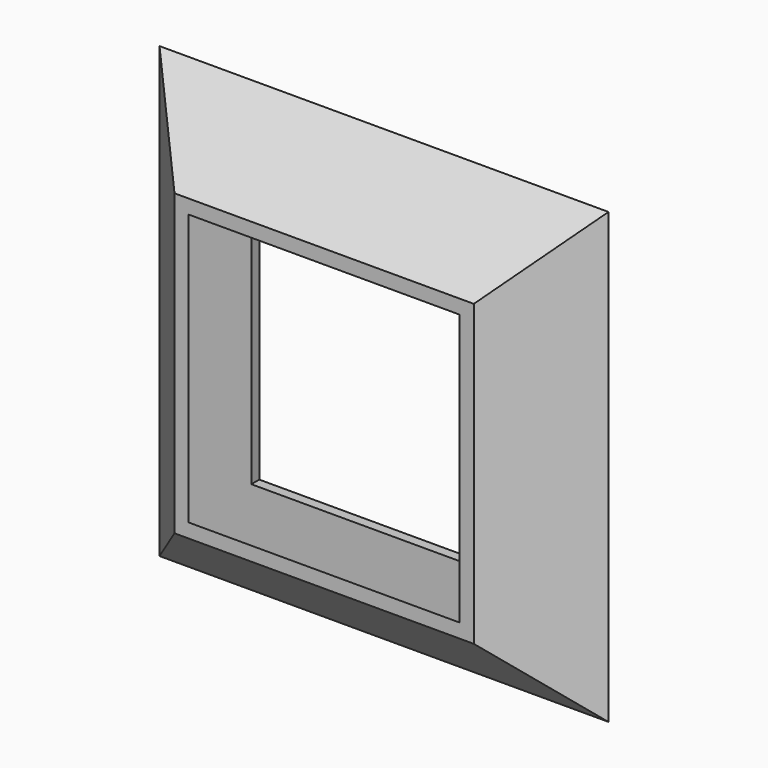
from build123d import *

# Parameters (mm, degrees)
F0_W        = 127
F0_H        = 127
F1_DEPTH    = 19.05
F2_T1_DEPTH = 257.6414957887
F2_T3_DEPTH = 257.6414957887
F3_T        = -2.54
F4_W        = 63.5
F4_H        = 63.5
F5_DEPTH    = 25.4


# Not quite as in the source:
# - a fillet or chamfer that OpenCascade refuses, or shapes differently, is made with other operations: its cross-section is extruded or revolved along the edge and cut away or added


with BuildPart() as f1:
    # F0 (on Front) → F1 (new body)
    with BuildSketch(Plane.XZ):
        with Locations((-51.5997745097, 45.6864875067)):
            Rectangle(F0_W, F0_H)
    extrude(amount=F1_DEPTH)

    # F2: chamfer of 25.4 on 4 edges, made by hand

    # F2_s2 → F2_t1 (cut)
    with BuildSketch(Plane.XY.offset(-83.1342603876)):
        Polygon((11.9002254903, 6.35), (-13.4997745097, -19.05), (11.9002254903, -19.05), align=None)
        Polygon((-115.0997745097, 6.35), (-89.6997745097, -19.05), (-115.0997745097, -19.05), align=None)
    extrude(amount=F2_T1_DEPTH, mode=Mode.SUBTRACT)

    # F2_s4 → F2_t3 (cut)
    with BuildSketch(Plane.YZ.offset(-180.420522404)):
        Polygon((6.35, 109.1864875067), (-19.05, 83.7864875067), (-19.05, 109.1864875067), align=None)
        Polygon((6.35, -17.8135124933), (-19.05, 7.5864875067), (-19.05, -17.8135124933), align=None)
    extrude(amount=F2_T3_DEPTH, mode=Mode.SUBTRACT)

    # F3
    f3_openings = [f1.faces().sort_by_distance(p)[0] for p in [
        (-51.599775, -19.05, 45.686488),
    ]]
    offset(amount=F3_T, openings=f3_openings, kind=Kind.INTERSECTION)

    # F4 (on face) → F5 (cut)
    with BuildSketch(Plane(origin=(0, 0, 0), x_dir=(-1, 0, 0), z_dir=(0, 1, 0))):
        with Locations((51.5997745097, 45.6864875067)):
            Rectangle(F4_W, F4_H)
    extrude(amount=-F5_DEPTH, mode=Mode.SUBTRACT)


solid = f1.part
